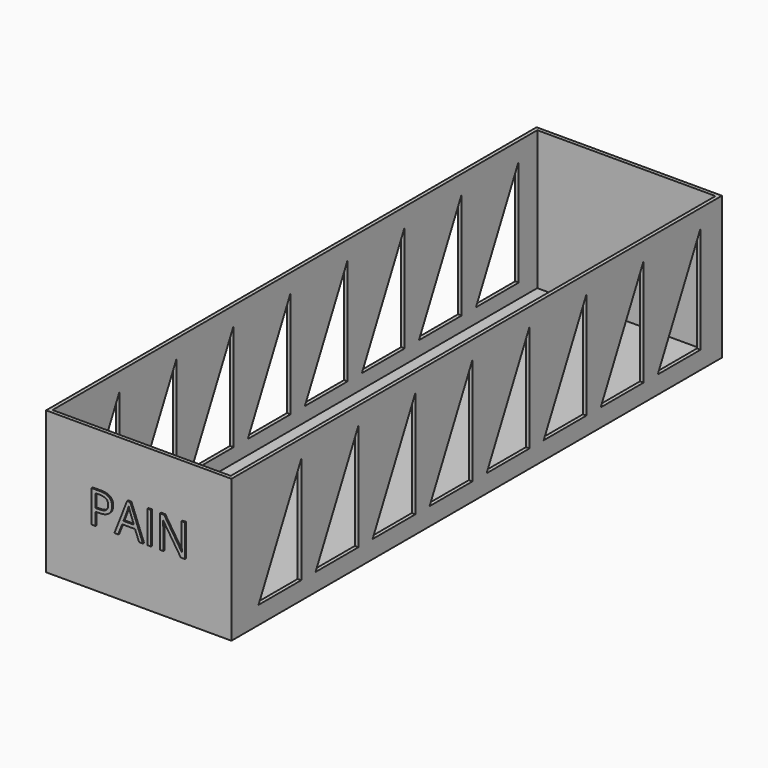
from build123d import *

# Parameters (mm, degrees)
F0_W         = 66.04
F0_H         = 218.44
F0_W_2       = 63.5
F0_H_2       = 215.9
F1_DEPTH     = 1.27
F2_DEPTH     = 50.8
F4_DEPTH     = 76.2
F5_TEXT_SIZE = 16.063092173
F6_DEPTH     = 0.508


# Not quite as in the source:
# - Text() gives the source's letters only with a copy of the font that has no kerning and outlines rounded to 1/6400 em; it was checked with that copy


with BuildPart() as f1:
    # F0 (on Top) → F1 (new body)
    with BuildSketch(Plane.XY):
        Rectangle(F0_W, F0_H)
        Rectangle(F0_W_2, F0_H_2, mode=Mode.SUBTRACT)
        Rectangle(F0_W_2, F0_H_2)
    extrude(amount=F1_DEPTH)

    # F0 (on Top) → F2 (join)
    with BuildSketch(Plane.XY):
        Rectangle(F0_W, F0_H)
        Rectangle(F0_W_2, F0_H_2, mode=Mode.SUBTRACT)
    extrude(amount=F2_DEPTH)

    # F3 (on face) → F4 (cut)
    with BuildSketch(Plane(origin=(-33.02, 0, 0), x_dir=(0, -1, 0), z_dir=(-1, 0, 0))):
        Polygon((-80.645, 6.35), (-99.695, 44.45), (-99.695, 6.35), align=None)
        Polygon((-74.295, 6.35), (-55.245, 6.35), (-74.295, 44.45), align=None)
        Polygon((-48.895, 6.35), (-29.845, 6.35), (-48.895, 44.45), align=None)
        Polygon((-23.495, 6.35), (-4.445, 6.35), (-23.495, 44.45), align=None)
        Polygon((1.905, 6.35), (20.955, 6.35), (1.905, 44.45), align=None)
        Polygon((27.305, 6.35), (46.355, 6.35), (27.305, 44.45), align=None)
        Polygon((52.705, 6.35), (71.755, 6.35), (52.705, 44.45), align=None)
        Polygon((78.105, 6.35), (97.155, 6.35), (78.105, 44.45), align=None)
    extrude(amount=-F4_DEPTH, mode=Mode.SUBTRACT)

    # F5 (on face) → F6 (join)
    with BuildSketch(Plane.XZ.offset(109.22)):
        with Locations((-17.9442308579, 20.5712914467)):
            Text('PAIN', F5_TEXT_SIZE, font='Open Sans', text_align=(TextAlign.LEFT, TextAlign.BOTTOM))
    extrude(amount=F6_DEPTH)


solid = f1.part
